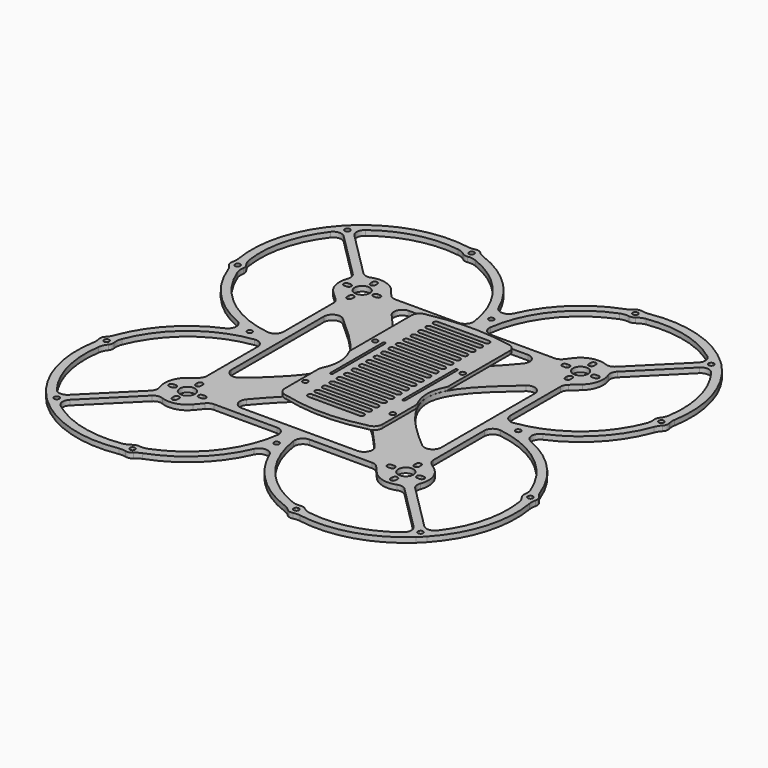
from build123d import *

# Parameters (mm, degrees)
F0_R     = 1.55
F0_R_2   = 4.5
F1_DEPTH = 3
F2_R     = 1.55
F3_DEPTH = 2
F5_DEPTH = 2


# Not quite as in the source:
# - a feature names something its author has since deleted; it is built from what else it names


with BuildPart() as f1:
    # F0 (on Top) → F1 (new body)
    with BuildSketch(Plane.XY):
        with BuildLine():
            ThreePointArc((4.5936412885, 90.9640892891), (1.5876e-06, 87.9385448385), (-4.5936380583, 90.9640893729))
            ThreePointArc((-4.5936380583, 90.9640893729), (-19.7997665524, 112.7493601662), (-42.3857157583, 126.7386155355))
            ThreePointArc((-42.3857157583, 126.7386155355), (-44.282976849, 127.6715883742), (-45.9416856044, 128.9825892242))
            ThreePointArc((-45.9416856044, 128.9825892242), (-47.711537449, 129.9897804476), (-49.7479021723, 129.9951119953))
            ThreePointArc((-49.7479021723, 129.9951119953), (-51.8387697531, 129.6815665856), (-53.9488258268, 129.814612931))
            ThreePointArc((-53.9488258268, 129.814612931), (-83.7536549239, 128.0187505985), (-109.6908840175, 113.2264179235))
            ThreePointArc((-109.6908840175, 113.2264179235), (-111.492270863, 111.492270863), (-113.2264179235, 109.6908840175))
            ThreePointArc((-113.2264179235, 109.6908840175), (-128.0187505985, 83.7536549239), (-129.814612931, 53.9488258268))
            ThreePointArc((-129.814612931, 53.9488258268), (-129.6815665856, 51.8387697531), (-129.9951119953, 49.7479021723))
            ThreePointArc((-129.9951119953, 49.7479021723), (-129.9897804476, 47.711537449), (-128.9825892242, 45.9416856044))
            ThreePointArc((-128.9825892242, 45.9416856044), (-127.6715883742, 44.282976849), (-126.7386155355, 42.3857157583))
            ThreePointArc((-126.7386155355, 42.3857157583), (-112.7493601662, 19.7997665524), (-90.9640893729, 4.5936380583))
            ThreePointArc((-90.9640893729, 4.5936380583), (-87.9385448385, -1.5876e-06), (-90.9640892891, -4.5936412885))
            ThreePointArc((-90.9640892891, -4.5936412885), (-112.7493564136, -19.7997669532), (-126.7386107311, -42.3857113668))
            ThreePointArc((-126.7386107311, -42.3857113668), (-127.6715848934, -44.2829742089), (-128.9825877652, -45.9416841141))
            ThreePointArc((-128.9825877652, -45.9416841141), (-129.9897804476, -47.711537449), (-129.9951114697, -49.7479041907))
            ThreePointArc((-129.9951114697, -49.7479041907), (-129.6815648767, -51.8387737737), (-129.8146109437, -53.9488320249))
            ThreePointArc((-129.8146109437, -53.9488320249), (-128.0187466409, -83.7536577022), (-113.2264144939, -109.6908833036))
            ThreePointArc((-113.2264144939, -109.6908833036), (-111.4922673823, -111.4922701), (-109.6908804846, -113.2264171062))
            ThreePointArc((-109.6908804846, -113.2264171062), (-83.7536558603, -128.018747189), (-53.9488320249, -129.8146109437))
            ThreePointArc((-53.9488320249, -129.8146109437), (-51.8387737737, -129.6815648767), (-49.7479041907, -129.9951114697))
            ThreePointArc((-49.7479041907, -129.9951114697), (-47.711537449, -129.9897804476), (-45.9416841141, -128.9825877652))
            ThreePointArc((-45.9416841141, -128.9825877652), (-44.2829742089, -127.6715848934), (-42.3857113668, -126.7386107311))
            ThreePointArc((-42.3857113668, -126.7386107311), (-19.7997655576, -112.7493550925), (-4.5936397708, -90.9640857581))
            ThreePointArc((-4.5936397708, -90.9640857581), (0, -87.938541039), (4.5936397708, -90.9640857581))
            ThreePointArc((4.5936397708, -90.9640857581), (19.7997655576, -112.7493550925), (42.3857113668, -126.7386107311))
            ThreePointArc((42.3857113668, -126.7386107311), (44.2829742089, -127.6715848934), (45.9416841141, -128.9825877652))
            ThreePointArc((45.9416841141, -128.9825877652), (47.711537449, -129.9897804476), (49.7479041907, -129.9951114697))
            ThreePointArc((49.7479041907, -129.9951114697), (51.8387737737, -129.6815648767), (53.9488320249, -129.8146109437))
            ThreePointArc((53.9488320249, -129.8146109437), (83.7536567813, -128.0187469149), (109.6908818941, -113.2264158001))
            ThreePointArc((109.6908818941, -113.2264158001), (111.4922687411, -111.4922687411), (113.2264158001, -109.6908818941))
            ThreePointArc((113.2264158001, -109.6908818941), (128.0187469149, -83.7536567813), (129.8146109437, -53.9488320249))
            ThreePointArc((129.8146109437, -53.9488320249), (129.6815648767, -51.8387737737), (129.9951114697, -49.7479041907))
            ThreePointArc((129.9951114697, -49.7479041907), (129.9897804476, -47.711537449), (128.9825877652, -45.9416841141))
            ThreePointArc((128.9825877652, -45.9416841141), (127.6715848934, -44.2829742089), (126.7386107311, -42.3857113668))
            ThreePointArc((126.7386107311, -42.3857113668), (112.7493550925, -19.7997655576), (90.9640857581, -4.5936397708))
            ThreePointArc((90.9640857581, -4.5936397708), (87.938541039, 0), (90.9640857581, 4.5936397708))
            ThreePointArc((90.9640857581, 4.5936397708), (112.7493550925, 19.7997655576), (126.7386107311, 42.3857113668))
            ThreePointArc((126.7386107311, 42.3857113668), (127.6715848934, 44.2829742089), (128.9825877652, 45.9416841141))
            ThreePointArc((128.9825877652, 45.9416841141), (129.9897804476, 47.711537449), (129.9951114697, 49.7479041907))
            ThreePointArc((129.9951114697, 49.7479041907), (129.6815648767, 51.8387737737), (129.8146109437, 53.9488320249))
            ThreePointArc((129.8146109437, 53.9488320249), (128.018747189, 83.7536558603), (113.2264171062, 109.6908804846))
            ThreePointArc((113.2264171062, 109.6908804846), (111.4922701, 111.4922673823), (109.6908833036, 113.2264144939))
            ThreePointArc((109.6908833036, 113.2264144939), (83.7536577022, 128.0187466408), (53.9488320249, 129.8146109437))
            ThreePointArc((53.9488320249, 129.8146109437), (51.8387737737, 129.6815648767), (49.7479041907, 129.9951114697))
            ThreePointArc((49.7479041907, 129.9951114697), (47.711537449, 129.9897804476), (45.9416841141, 128.9825877652))
            ThreePointArc((45.9416841141, 128.9825877652), (44.2829742089, 127.6715848934), (42.3857113668, 126.7386107311))
            ThreePointArc((42.3857113668, 126.7386107311), (19.7997669532, 112.7493564136), (4.5936412885, 90.9640892891))
        make_face()
        with Locations((-108.2905437355, -108.153230011)):
            Circle(F0_R, mode=Mode.SUBTRACT)
        with Locations((-48.7398474892, -126.1242172983)):
            Circle(F0_R, mode=Mode.SUBTRACT)
        with BuildLine():
            Line((-66.5, -74.5), (-66.5, -73))
            ThreePointArc((-66.5, -73), (-65, -71.5), (-63.5, -73))
            Line((-63.5, -73), (-63.5, -74.5))
            ThreePointArc((-63.5, -74.5), (-65, -76), (-66.5, -74.5))
        make_face(mode=Mode.SUBTRACT)
        with Locations((-126.1242172983, -48.7398474892)):
            Circle(F0_R, mode=Mode.SUBTRACT)
        with BuildLine():
            Line((-73, -66.5), (-74.5, -66.5))
            ThreePointArc((-74.5, -66.5), (-76, -65), (-74.5, -63.5))
            Line((-74.5, -63.5), (-73, -63.5))
            ThreePointArc((-73, -63.5), (-71.5, -65), (-73, -66.5))
        make_face(mode=Mode.SUBTRACT)
        with Locations((-79.8885448385, 0)):
            Circle(F0_R, mode=Mode.SUBTRACT)
        with Locations((-65, -65)):
            Circle(F0_R_2, mode=Mode.SUBTRACT)
        with BuildLine():
            ThreePointArc((-57, -66.5), (-58.5, -65), (-57, -63.5))
            Line((-57, -63.5), (-55.5, -63.5))
            ThreePointArc((-55.5, -63.5), (-54, -65), (-55.5, -66.5))
            Line((-55.5, -66.5), (-57, -66.5))
        make_face(mode=Mode.SUBTRACT)
        with BuildLine():
            Line((-66.5, -57), (-66.5, -55.5))
            ThreePointArc((-66.5, -55.5), (-65, -54), (-63.5, -55.5))
            Line((-63.5, -55.5), (-63.5, -57))
            ThreePointArc((-63.5, -57), (-65, -58.5), (-66.5, -57))
        make_face(mode=Mode.SUBTRACT)
        with Locations((48.7398474892, -126.1242172983)):
            Circle(F0_R, mode=Mode.SUBTRACT)
        with Locations((0, -79.8885448385)):
            Circle(F0_R, mode=Mode.SUBTRACT)
        with BuildLine():
            ThreePointArc((66.5, -74.5), (65, -76), (63.5, -74.5))
            Line((63.5, -74.5), (63.5, -73))
            ThreePointArc((63.5, -73), (65, -71.5), (66.5, -73))
            Line((66.5, -73), (66.5, -74.5))
        make_face(mode=Mode.SUBTRACT)
        with Locations((108.2784277556, -108.1560280507)):
            Circle(F0_R, mode=Mode.SUBTRACT)
        with BuildLine():
            ThreePointArc((57, -63.5), (58.5, -65), (57, -66.5))
            Line((57, -66.5), (55.5, -66.5))
            ThreePointArc((55.5, -66.5), (54, -65), (55.5, -63.5))
            Line((55.5, -63.5), (57, -63.5))
        make_face(mode=Mode.SUBTRACT)
        with Locations((65, -65)):
            Circle(F0_R_2, mode=Mode.SUBTRACT)
        with BuildLine():
            ThreePointArc((66.5, -57), (65, -58.5), (63.5, -57))
            Line((63.5, -57), (63.5, -55.5))
            ThreePointArc((63.5, -55.5), (65, -54), (66.5, -55.5))
            Line((66.5, -55.5), (66.5, -57))
        make_face(mode=Mode.SUBTRACT)
        with BuildLine():
            ThreePointArc((-78.7260276961, 75.1904937901), (-77.3700677078, 72.6909557736), (-77.5962746825, 69.8563220777))
            ThreePointArc((-77.5962746825, 69.8563220777), (-78.1774623607, 62.066659629), (-74.3468847944, 55.2590685948))
            ThreePointArc((-74.3468847944, 55.2590685948), (-55.8574100489, 55.0670724866), (-54.5192604238, 73.5090597562))
            ThreePointArc((-54.5192604238, 73.5090597562), (-61.5236729853, 78.0447365051), (-69.8563220777, 77.5962746825))
            ThreePointArc((-69.8563220777, 77.5962746825), (-72.6909557736, 77.3700677078), (-75.1904937901, 78.7260276961))
            Line((-75.1904937901, 78.7260276961), (-102.2950830455, 105.8306169514))
            ThreePointArc((-102.2950830455, 105.8306169514), (-103.7481732445, 109.7032406669), (-101.7873113942, 113.3451778401))
            ThreePointArc((-101.7873113942, 113.3451778401), (-80.0827992563, 123.8478688365), (-56.0022199647, 125.0799671641))
            ThreePointArc((-56.0022199647, 125.0799671641), (-53.4825995412, 124.3550905641), (-51.2379870694, 123.0002296802))
            ThreePointArc((-51.2379870694, 123.0002296802), (-49.7681575294, 122.258654149), (-48.1241365653, 122.1718888632))
            ThreePointArc((-48.1241365653, 122.1718888632), (-45.5030157293, 122.2323762703), (-42.9562600942, 121.6095047758))
            ThreePointArc((-42.9562600942, 121.6095047758), (-17.2773803845, 102.5914096175), (-4.8022395632, 73.1726457399))
            ThreePointArc((-4.8022395632, 73.1726457399), (-5.9909393236, 69.2108685569), (-9.7567877473, 67.5))
            Line((-9.7567877473, 67.5), (-47.2749619701, 67.5))
            ThreePointArc((-47.2749619701, 67.5), (-49.4332948043, 67.989833775), (-51.1687379105, 69.3633602493))
            add(Edge.make_bspline(
                [(-51.1687379105, 69.3633602493), (-47.007111135, 64.1971813129), (-42.9204896878, 59.0857782526), (-38.8861434054, 54.2837422746)],
                knots=[0.0293673697, 0.0293673697, 0.0293673697, 0.0293673697, 0.1393383892, 0.1393383892, 0.1393383892, 0.1393383892], degree=3))
            ThreePointArc((-38.8861434054, 54.2837422746), (-39.5900475875, 59.6117186571), (-35.0578688274, 62.5))
            Line((-35.0578688274, 62.5), (35.6142056633, 62.5))
            ThreePointArc((35.6142056633, 62.5), (40.1396288907, 59.6261572409), (39.4629102085, 54.3082178452))
            add(Edge.make_bspline(
                [(39.4629102085, 54.3082178452), (43.4572386204, 59.1246461501), (47.4477718972, 64.2594353508), (51.4265936274, 69.4628891406)],
                knots=[0.8640600007, 0.8640600007, 0.8640600007, 0.8640600007, 0.9739367654, 0.9739367654, 0.9739367654, 0.9739367654], degree=3))
            ThreePointArc((51.4265936274, 69.4628891406), (49.6699228907, 68.0175032461), (47.4546976535, 67.5))
            Line((47.4546976535, 67.5), (9.7567877473, 67.5))
            ThreePointArc((9.7567877473, 67.5), (5.9909393236, 69.2108685569), (4.8022395632, 73.1726457399))
            ThreePointArc((4.8022395632, 73.1726457399), (17.2773803845, 102.5914096175), (42.9562600942, 121.6095047758))
            ThreePointArc((42.9562600942, 121.6095047758), (45.5030157293, 122.2323762703), (48.1241365653, 122.1718888632))
            ThreePointArc((48.1241365653, 122.1718888632), (49.7681575294, 122.258654149), (51.2379870694, 123.0002296802))
            ThreePointArc((51.2379870694, 123.0002296802), (53.4825995412, 124.3550905641), (56.0022199647, 125.0799671641))
            ThreePointArc((56.0022199647, 125.0799671641), (80.0828001163, 123.8478686161), (101.7873128072, 113.3451767649))
            ThreePointArc((101.7873128072, 113.3451767649), (103.748174551, 109.7032395344), (102.2950842388, 105.8306158614))
            Line((102.2950842388, 105.8306158614), (75.1904941913, 78.7260273982))
            ThreePointArc((75.1904941913, 78.7260273982), (72.6909561352, 77.370067483), (69.8563224458, 77.5962745406))
            ThreePointArc((69.8563224458, 77.5962745406), (61.3181994895, 77.9882387182), (54.2558912586, 73.1739909073))
            ThreePointArc((54.2558912586, 73.1739909073), (55.8750675797, 55.0508488641), (74.0703287451, 55.0010432317))
            ThreePointArc((74.0703287451, 55.0010432317), (78.1350771686, 61.8823489971), (77.5962748245, 69.8563217095))
            ThreePointArc((77.5962748245, 69.8563217095), (77.3700679326, 72.6909554121), (78.7260279939, 75.190493389))
            Line((78.7260279939, 75.190493389), (105.8306180414, 102.2950818521))
            ThreePointArc((105.8306180414, 102.2950818521), (109.7032417994, 103.7481719379), (113.3451789152, 101.7873099812))
            ThreePointArc((113.3451789152, 101.7873099812), (123.8478690569, 80.0827983963), (125.0799671641, 56.0022199647))
            ThreePointArc((125.0799671641, 56.0022199647), (124.3550905641, 53.4825995412), (123.0002296802, 51.2379870694))
            ThreePointArc((123.0002296802, 51.2379870694), (122.258654149, 49.7681575294), (122.1718888632, 48.1241365653))
            ThreePointArc((122.1718888632, 48.1241365653), (122.2323762703, 45.5030157293), (121.6095047758, 42.9562600942))
            ThreePointArc((121.6095047758, 42.9562600942), (102.5914096175, 17.2773803845), (73.1726457399, 4.8022395632))
            ThreePointArc((73.1726457399, 4.8022395632), (69.2108685569, 5.9909393236), (67.5, 9.7567877473))
            Line((67.5, 9.7567877473), (67.5, 46.9024650002))
            ThreePointArc((67.5, 46.9024650002), (67.9450696625, 48.9646506418), (69.2010438482, 50.6597097764))
            add(Edge.make_bspline(
                [(69.2010438482, 50.6597097764), (64.0951140729, 46.1765740091), (59.0182901872, 41.9052788751), (54.2353248312, 37.7820833857)],
                knots=[0.0348728398, 0.0348728398, 0.0348728398, 0.0348728398, 0.1445829675, 0.1445829675, 0.1445829675, 0.1445829675], degree=3))
            ThreePointArc((54.2353248312, 37.7820833857), (59.5828615119, 38.5405267444), (62.5, 33.9950138006))
            Line((62.5, 33.9950138006), (62.5, -35.5495988309))
            ThreePointArc((62.5, -35.5495988309), (59.6206264771, -40.0776164264), (54.2988226622, -39.3904924316))
            add(Edge.make_bspline(
                [(54.2988226622, -39.3904924316), (59.1121784473, -43.4021644694), (64.2467475497, -47.4153572737), (69.4560669959, -51.4128712838)],
                knots=[0.8650150287, 0.8650150287, 0.8650150287, 0.8650150287, 0.9740421792, 0.9740421792, 0.9740421792, 0.9740421792], degree=3))
            ThreePointArc((69.4560669959, -51.4128712838), (68.0156012097, -49.6575734697), (67.5, -47.4462011605))
            Line((67.5, -47.4462011605), (67.5, -9.7567877473))
            ThreePointArc((67.5, -9.7567877473), (69.2108685569, -5.9909393236), (73.1726457399, -4.8022395632))
            ThreePointArc((73.1726457399, -4.8022395632), (102.5914096175, -17.2773803845), (121.6095047758, -42.9562600942))
            ThreePointArc((121.6095047758, -42.9562600942), (122.2323762703, -45.5030157293), (122.1718888632, -48.1241365653))
            ThreePointArc((122.1718888632, -48.1241365653), (122.258654149, -49.7681575294), (123.0002296802, -51.2379870694))
            ThreePointArc((123.0002296802, -51.2379870694), (124.3550905641, -53.4825995412), (125.0799671641, -56.0022199647))
            ThreePointArc((125.0799671641, -56.0022199647), (123.8478688365, -80.0827992563), (113.3451778401, -101.7873113942))
            ThreePointArc((113.3451778401, -101.7873113942), (109.7032406669, -103.7481732445), (105.8306169514, -102.2950830455))
            Line((105.8306169514, -102.2950830455), (78.7260276961, -75.1904937901))
            ThreePointArc((78.7260276961, -75.1904937901), (77.3700677078, -72.6909557736), (77.5962746825, -69.8563220777))
            ThreePointArc((77.5962746825, -69.8563220777), (77.9903375994, -61.3256117442), (73.1862480092, -54.2652273647))
            ThreePointArc((73.1862480092, -54.2652273647), (55.0961710642, -55.8258966427), (54.9219208197, -73.9823337745))
            ThreePointArc((54.9219208197, -73.9823337745), (61.8248103944, -78.1212869403), (69.8563220777, -77.5962746825))
            ThreePointArc((69.8563220777, -77.5962746825), (72.6909557736, -77.3700677078), (75.1904937901, -78.7260276961))
            Line((75.1904937901, -78.7260276961), (102.2950830455, -105.8306169514))
            ThreePointArc((102.2950830455, -105.8306169514), (103.7481732445, -109.7032406669), (101.7873113942, -113.3451778401))
            ThreePointArc((101.7873113942, -113.3451778401), (80.0827992563, -123.8478688365), (56.0022199647, -125.0799671641))
            ThreePointArc((56.0022199647, -125.0799671641), (53.4825995412, -124.3550905641), (51.2379870694, -123.0002296802))
            ThreePointArc((51.2379870694, -123.0002296802), (49.7681575294, -122.258654149), (48.1241365653, -122.1718888632))
            ThreePointArc((48.1241365653, -122.1718888632), (45.5030157293, -122.2323762703), (42.9562600942, -121.6095047758))
            ThreePointArc((42.9562600942, -121.6095047758), (17.2773803845, -102.5914096175), (4.8022395632, -73.1726457399))
            ThreePointArc((4.8022395632, -73.1726457399), (5.9909393236, -69.2108685569), (9.7567877473, -67.5))
            Line((9.7567877473, -67.5), (46.9610754937, -67.5))
            ThreePointArc((46.9610754937, -67.5), (49.0351777215, -67.9504835478), (50.7355403773, -69.2207600206))
            add(Edge.make_bspline(
                [(50.7355403773, -69.2207600206), (46.2776004608, -64.0895900624), (42.0082462932, -59.0081310929), (37.8793761718, -54.2306155101)],
                knots=[0.0336445481, 0.0336445481, 0.0336445481, 0.0336445481, 0.1425668185, 0.1425668185, 0.1425668185, 0.1425668185], degree=3))
            ThreePointArc((37.8793761718, -54.2306155101), (38.6431792121, -59.5800333592), (34.0963714061, -62.5))
            Line((34.0963714061, -62.5), (-34.6716965747, -62.5))
            ThreePointArc((-34.6716965747, -62.5), (-39.2116462302, -59.594959934), (-38.4761016269, -54.25554285))
            add(Edge.make_bspline(
                [(-38.4761016269, -54.25554285), (-42.5524815665, -59.0354489236), (-46.7247402937, -64.1334390375), (-51.0163929038, -69.3081210856)],
                knots=[0.86152407, 0.86152407, 0.86152407, 0.86152407, 0.9696650908, 0.9696650908, 0.9696650908, 0.9696650908], degree=3))
            ThreePointArc((-51.0163929038, -69.3081210856), (-49.2938689584, -67.974550046), (-47.1677686047, -67.5))
            Line((-47.1677686047, -67.5), (-9.7567877474, -67.5))
            ThreePointArc((-9.7567877474, -67.5), (-5.9909393237, -69.2108685569), (-4.8022395633, -73.1726457399))
            ThreePointArc((-4.8022395633, -73.1726457399), (-17.2773803846, -102.5914096175), (-42.9562600944, -121.6095047758))
            ThreePointArc((-42.9562600944, -121.6095047758), (-45.5030157294, -122.2323762703), (-48.1241365654, -122.1718888632))
            ThreePointArc((-48.1241365654, -122.1718888632), (-49.7681575294, -122.258654149), (-51.2379870693, -123.0002296802))
            ThreePointArc((-51.2379870693, -123.0002296802), (-53.4825995411, -124.355090564), (-56.0022199645, -125.079967164))
            ThreePointArc((-56.0022199645, -125.079967164), (-80.0827983962, -123.8478690568), (-101.7873099811, -113.3451789152))
            ThreePointArc((-101.7873099811, -113.3451789152), (-103.7481719378, -109.7032417994), (-102.295081852, -105.8306180414))
            Line((-102.295081852, -105.8306180414), (-75.190493389, -78.7260279939))
            ThreePointArc((-75.190493389, -78.7260279939), (-72.6909554121, -77.3700679326), (-69.8563217095, -77.5962748245))
            ThreePointArc((-69.8563217095, -77.5962748245), (-61.6280970797, -78.0721180647), (-54.6566830252, -73.6755860873))
            ThreePointArc((-54.6566830252, -73.6755860873), (-55.3115936341, -55.5986818962), (-73.3606290294, -54.4004772639))
            ThreePointArc((-73.3606290294, -54.4004772639), (-78.019936228, -61.431910789), (-77.5962745406, -69.8563224458))
            ThreePointArc((-77.5962745406, -69.8563224458), (-77.370067483, -72.6909561352), (-78.7260273982, -75.1904941913))
            Line((-78.7260273982, -75.1904941913), (-105.8306158613, -102.2950842388))
            ThreePointArc((-105.8306158613, -102.2950842388), (-109.7032395344, -103.7481745509), (-113.3451767648, -101.7873128071))
            ThreePointArc((-113.3451767648, -101.7873128071), (-123.847868616, -80.0828001162), (-125.079967164, -56.0022199645))
            ThreePointArc((-125.079967164, -56.0022199645), (-124.355090564, -53.4825995411), (-123.0002296802, -51.2379870693))
            ThreePointArc((-123.0002296802, -51.2379870693), (-122.258654149, -49.7681575294), (-122.1718888632, -48.1241365654))
            ThreePointArc((-122.1718888632, -48.1241365654), (-122.2323762703, -45.5030157294), (-121.6095047758, -42.9562600944))
            ThreePointArc((-121.6095047758, -42.9562600944), (-102.5915462524, -17.277488013), (-73.1729904451, -4.8022863626))
            ThreePointArc((-73.1729904451, -4.8022863626), (-69.2111956733, -5.9909728541), (-67.5003163344, -9.7568306947))
            Line((-67.5003163344, -9.7568306947), (-67.5003163328, -47.353236691))
            ThreePointArc((-67.5003163328, -47.353236691), (-68.0006204029, -49.5333138774), (-69.4014109482, -51.2771104681))
            add(Edge.make_bspline(
                [(-54.2790618736, -39.0485616103), (-59.0828616964, -43.094423634), (-64.2057413604, -47.1737958924), (-69.4014109482, -51.2771104681)],
                knots=[0.8641405018, 0.8641405018, 0.8641405018, 0.8641405018, 0.9725362801, 0.9725362801, 0.9725362801, 0.9725362801], degree=3))
            ThreePointArc((-54.2790618736, -39.0485616103), (-59.6089463445, -39.7576935316), (-62.5, -35.2242240748))
            Line((-62.5, -35.2242240748), (-62.5, 33.4095018987))
            ThreePointArc((-62.5, 33.4095018987), (-59.5674116994, 37.9620625919), (-54.209676454, 37.1743087945))
            add(Edge.make_bspline(
                [(-69.1233391423, 50.3680202269), (-64.0476785875, 45.7195000527), (-58.9859996351, 41.3486659558), (-54.209676454, 37.1743087945)],
                knots=[0.0376140132, 0.0376140132, 0.0376140132, 0.0376140132, 0.147134592, 0.147134592, 0.147134592, 0.147134592], degree=3))
            ThreePointArc((-69.1233391423, 50.3680202269), (-67.9240249358, 48.6950792761), (-67.5003163367, 46.6807414163))
            Line((-67.5003163367, 46.6807414163), (-67.5003163352, 9.7568306951))
            ThreePointArc((-67.5003163352, 9.7568306951), (-69.211195674, 5.9909728542), (-73.1729904459, 4.8022863626))
            ThreePointArc((-73.1729904459, 4.8022863626), (-102.5915462527, 17.2774880132), (-121.6095047758, 42.9562600942))
            ThreePointArc((-121.6095047758, 42.9562600942), (-122.2323762703, 45.5030157293), (-122.1718888632, 48.1241365653))
            ThreePointArc((-122.1718888632, 48.1241365653), (-122.258654149, 49.7681575294), (-123.0002296802, 51.2379870694))
            ThreePointArc((-123.0002296802, 51.2379870694), (-124.3550905641, 53.4825995412), (-125.0799671641, 56.0022199647))
            ThreePointArc((-125.0799671641, 56.0022199647), (-123.8478688365, 80.0827992563), (-113.3451778401, 101.7873113942))
            ThreePointArc((-113.3451778401, 101.7873113942), (-109.7032406669, 103.7481732445), (-105.8306169514, 102.2950830455))
            Line((-105.8306169514, 102.2950830455), (-78.7260276961, 75.1904937901))
        make_face(mode=Mode.SUBTRACT)
        with BuildLine():
            ThreePointArc((74.5, -63.5), (76, -65), (74.5, -66.5))
            Line((74.5, -66.5), (73, -66.5))
            ThreePointArc((73, -66.5), (71.5, -65), (73, -63.5))
            Line((73, -63.5), (74.5, -63.5))
        make_face(mode=Mode.SUBTRACT)
        with Locations((126.1242172983, -48.7398474892)):
            Circle(F0_R, mode=Mode.SUBTRACT)
        with Locations((79.8885448385, 0)):
            Circle(F0_R, mode=Mode.SUBTRACT)
        with Locations((-126.1242172983, 48.7398474892)):
            Circle(F0_R, mode=Mode.SUBTRACT)
        with BuildLine():
            ThreePointArc((-73, 66.5), (-71.5, 65), (-73, 63.5))
            Line((-73, 63.5), (-74.5, 63.5))
            ThreePointArc((-74.5, 63.5), (-76, 65), (-74.5, 66.5))
            Line((-74.5, 66.5), (-73, 66.5))
        make_face(mode=Mode.SUBTRACT)
        with BuildLine():
            ThreePointArc((-63.5, 55.5), (-65, 54), (-66.5, 55.5))
            Line((-66.5, 55.5), (-66.5, 57))
            ThreePointArc((-66.5, 57), (-65, 58.5), (-63.5, 57))
            Line((-63.5, 57), (-63.5, 55.5))
        make_face(mode=Mode.SUBTRACT)
        with Locations((-65, 65)):
            Circle(F0_R_2, mode=Mode.SUBTRACT)
        with BuildLine():
            Line((-55.5, 63.5), (-57, 63.5))
            ThreePointArc((-57, 63.5), (-58.5, 65), (-57, 66.5))
            Line((-57, 66.5), (-55.5, 66.5))
            ThreePointArc((-55.5, 66.5), (-54, 65), (-55.5, 63.5))
        make_face(mode=Mode.SUBTRACT)
        with Locations((-108.3014905595, 108.1507019099)):
            Circle(F0_R, mode=Mode.SUBTRACT)
        with BuildLine():
            ThreePointArc((-63.5, 73), (-65, 71.5), (-66.5, 73))
            Line((-66.5, 73), (-66.5, 74.5))
            ThreePointArc((-66.5, 74.5), (-65, 76), (-63.5, 74.5))
            Line((-63.5, 74.5), (-63.5, 73))
        make_face(mode=Mode.SUBTRACT)
        with Locations((-48.7398474892, 126.1242172983)):
            Circle(F0_R, mode=Mode.SUBTRACT)
        with BuildLine():
            Line((63.5, 55.5), (63.5, 57))
            ThreePointArc((63.5, 57), (65, 58.5), (66.5, 57))
            Line((66.5, 57), (66.5, 55.5))
            ThreePointArc((66.5, 55.5), (65, 54), (63.5, 55.5))
        make_face(mode=Mode.SUBTRACT)
        with BuildLine():
            Line((55.5, 66.5), (57, 66.5))
            ThreePointArc((57, 66.5), (58.5, 65), (57, 63.5))
            Line((57, 63.5), (55.5, 63.5))
            ThreePointArc((55.5, 63.5), (54, 65), (55.5, 66.5))
        make_face(mode=Mode.SUBTRACT)
        with Locations((65, 65)):
            Circle(F0_R_2, mode=Mode.SUBTRACT)
        with BuildLine():
            Line((74.5, 63.5), (73, 63.5))
            ThreePointArc((73, 63.5), (71.5, 65), (73, 66.5))
            Line((73, 66.5), (74.5, 66.5))
            ThreePointArc((74.5, 66.5), (76, 65), (74.5, 63.5))
        make_face(mode=Mode.SUBTRACT)
        with Locations((126.1242172983, 48.7398474892)):
            Circle(F0_R, mode=Mode.SUBTRACT)
        with Locations((0, 79.8885448385)):
            Circle(F0_R, mode=Mode.SUBTRACT)
        with BuildLine():
            Line((66.5, 74.5), (66.5, 73))
            ThreePointArc((66.5, 73), (65, 71.5), (63.5, 73))
            Line((63.5, 73), (63.5, 74.5))
            ThreePointArc((63.5, 74.5), (65, 76), (66.5, 74.5))
        make_face(mode=Mode.SUBTRACT)
        with Locations((48.7398474892, 126.1242172983)):
            Circle(F0_R, mode=Mode.SUBTRACT)
        with Locations((108.153230011, 108.2905437356)):
            Circle(F0_R, mode=Mode.SUBTRACT)
        with BuildLine():
            ThreePointArc((-54.5192604238, 73.5090597562), (-55.8574100489, 55.0670724866), (-74.3468847944, 55.2590685948))
            add(Edge.make_bspline(
                [(-74.3468847944, 55.2590685948), (-72.6113826473, 53.5937721304), (-70.8665363109, 51.9645192675), (-69.1233391423, 50.3680202269)],
                knots=[0, 0, 0, 0, 0.0376140132, 0.0376140132, 0.0376140132, 0.0376140132], degree=3))
            add(Edge.make_bspline(
                [(-69.1233391423, 50.3680202269), (-64.0476785875, 45.7195000527), (-58.9859996351, 41.3486659558), (-54.209676454, 37.1743087945)],
                knots=[0.0376140132, 0.0376140132, 0.0376140132, 0.0376140132, 0.147134592, 0.147134592, 0.147134592, 0.147134592], degree=3))
            add(Edge.make_bspline(
                [(-54.209676454, 37.1743087945), (-38.7237596273, 23.6401015491), (-13.5112663594, 0.4819895204), (-38.2399723309, -25.540100461), (-54.2790618736, -39.0485616103)],
                knots=[0.147134592, 0.147134592, 0.147134592, 0.147134592, 0.5022250058, 0.8641405018, 0.8641405018, 0.8641405018, 0.8641405018], degree=3))
            add(Edge.make_bspline(
                [(-54.2790618736, -39.0485616103), (-59.0828616964, -43.094423634), (-64.2057413604, -47.1737958924), (-69.4014109482, -51.2771104681)],
                knots=[0.8641405018, 0.8641405018, 0.8641405018, 0.8641405018, 0.9725362801, 0.9725362801, 0.9725362801, 0.9725362801], degree=3))
            add(Edge.make_bspline(
                [(-69.4014109482, -51.2771104681), (-70.7178128987, -52.3167476543), (-72.0388875207, -53.3579217921), (-73.3606290294, -54.4004772639)],
                knots=[0.9725362801, 0.9725362801, 0.9725362801, 0.9725362801, 1, 1, 1, 1], degree=3))
            ThreePointArc((-73.3606290294, -54.4004772639), (-55.3115936341, -55.5986818962), (-54.6566830252, -73.6755860873))
            add(Edge.make_bspline(
                [(-51.0163929038, -69.3081210856), (-52.2202551514, -70.7596841376), (-53.4335121775, -72.2172818685), (-54.6566830252, -73.6755860873)],
                knots=[0.9696650908, 0.9696650908, 0.9696650908, 0.9696650908, 1, 1, 1, 1], degree=3))
            add(Edge.make_bspline(
                [(-38.4761016269, -54.25554285), (-42.5524815665, -59.0354489236), (-46.7247402937, -64.1334390375), (-51.0163929038, -69.3081210856)],
                knots=[0.86152407, 0.86152407, 0.86152407, 0.86152407, 0.9696650908, 0.9696650908, 0.9696650908, 0.9696650908], degree=3))
            add(Edge.make_bspline(
                [(37.8793761718, -54.2306155101), (24.3041480834, -38.5227192032), (0.0997442999, -13.5842522629), (-24.8744525972, -38.3064395346), (-38.4761016269, -54.25554285)],
                knots=[0.1425668185, 0.1425668185, 0.1425668185, 0.1425668185, 0.500690136, 0.86152407, 0.86152407, 0.86152407, 0.86152407], degree=3))
            add(Edge.make_bspline(
                [(50.7355403773, -69.2207600206), (46.2776004608, -64.0895900624), (42.0082462932, -59.0081310929), (37.8793761718, -54.2306155101)],
                knots=[0.0336445481, 0.0336445481, 0.0336445481, 0.0336445481, 0.1425668185, 0.1425668185, 0.1425668185, 0.1425668185], degree=3))
            add(Edge.make_bspline(
                [(54.9219208197, -73.9823337745), (53.5075225493, -72.3953945536), (52.112534936, -70.8057058127), (50.7355403773, -69.2207600206)],
                knots=[0, 0, 0, 0, 0.0336445481, 0.0336445481, 0.0336445481, 0.0336445481], degree=3))
            ThreePointArc((54.9219208197, -73.9823337745), (55.0961710642, -55.8258966427), (73.1862480092, -54.2652273647))
            add(Edge.make_bspline(
                [(69.4560669959, -51.4128712838), (70.6963321973, -52.3646227688), (71.940834612, -53.3154855034), (73.1862480092, -54.2652273647)],
                knots=[0.9740421792, 0.9740421792, 0.9740421792, 0.9740421792, 1, 1, 1, 1], degree=3))
            add(Edge.make_bspline(
                [(54.2988226622, -39.3904924316), (59.1121784473, -43.4021644694), (64.2467475497, -47.4153572737), (69.4560669959, -51.4128712838)],
                knots=[0.8650150287, 0.8650150287, 0.8650150287, 0.8650150287, 0.9740421792, 0.9740421792, 0.9740421792, 0.9740421792], degree=3))
            add(Edge.make_bspline(
                [(54.2353248312, 37.7820833857), (38.6550415809, 24.3509692464), (13.5326368893, 0.4431862355), (38.2705199865, -26.0317679723), (54.2988226622, -39.3904924316)],
                knots=[0.1445829675, 0.1445829675, 0.1445829675, 0.1445829675, 0.5019585155, 0.8650150287, 0.8650150287, 0.8650150287, 0.8650150287], degree=3))
            add(Edge.make_bspline(
                [(69.2010438482, 50.6597097764), (64.0951140729, 46.1765740091), (59.0182901872, 41.9052788751), (54.2353248312, 37.7820833857)],
                knots=[0.0348728398, 0.0348728398, 0.0348728398, 0.0348728398, 0.1445829675, 0.1445829675, 0.1445829675, 0.1445829675], degree=3))
            add(Edge.make_bspline(
                [(74.0703287451, 55.0010432317), (72.4499615375, 53.5311635631), (70.8240323045, 52.0847347804), (69.2010438482, 50.6597097764)],
                knots=[0, 0, 0, 0, 0.0348728398, 0.0348728398, 0.0348728398, 0.0348728398], degree=3))
            ThreePointArc((74.0703287451, 55.0010432317), (55.8750675797, 55.0508488641), (54.2558912586, 73.1739909073))
            add(Edge.make_bspline(
                [(51.4265936274, 69.4628891406), (52.3703870168, 70.6971704484), (53.3135214459, 71.9353152278), (54.2558912586, 73.1739909073)],
                knots=[0.9739367654, 0.9739367654, 0.9739367654, 0.9739367654, 1, 1, 1, 1], degree=3))
            add(Edge.make_bspline(
                [(39.4629102085, 54.3082178452), (43.4572386204, 59.1246461501), (47.4477718972, 64.2594353508), (51.4265936274, 69.4628891406)],
                knots=[0.8640600007, 0.8640600007, 0.8640600007, 0.8640600007, 0.9739367654, 0.9739367654, 0.9739367654, 0.9739367654], degree=3))
            add(Edge.make_bspline(
                [(-38.8861434054, 54.2837422746), (-25.628452755, 38.5032655801), (-0.1737443139, 13.5570975552), (26.2546916853, 38.3815260478), (39.4629102085, 54.3082178452)],
                knots=[0.1393383892, 0.1393383892, 0.1393383892, 0.1393383892, 0.5007257504, 0.8640600007, 0.8640600007, 0.8640600007, 0.8640600007], degree=3))
            add(Edge.make_bspline(
                [(-51.1687379105, 69.3633602493), (-47.007111135, 64.1971813129), (-42.9204896878, 59.0857782526), (-38.8861434054, 54.2837422746)],
                knots=[0.0293673697, 0.0293673697, 0.0293673697, 0.0293673697, 0.1393383892, 0.1393383892, 0.1393383892, 0.1393383892], degree=3))
            add(Edge.make_bspline(
                [(-54.5192604238, 73.5090597562), (-53.3967820872, 72.126485951), (-52.2800855412, 70.7429699621), (-51.1687379105, 69.3633602493)],
                knots=[0, 0, 0, 0, 0.0293673697, 0.0293673697, 0.0293673697, 0.0293673697], degree=3))
        make_face()
        with Locations((-26, -26)):
            Circle(F0_R, mode=Mode.SUBTRACT)
        with Locations((-15.25, -15.25)):
            Circle(F0_R, mode=Mode.SUBTRACT)
        with Locations((26, -26)):
            Circle(F0_R, mode=Mode.SUBTRACT)
        with Locations((15.25, -15.25)):
            Circle(F0_R, mode=Mode.SUBTRACT)
        with Locations((-15.25, 15.25)):
            Circle(F0_R, mode=Mode.SUBTRACT)
        with Locations((-26, 26)):
            Circle(F0_R, mode=Mode.SUBTRACT)
        with Locations((15.25, 15.25)):
            Circle(F0_R, mode=Mode.SUBTRACT)
        with Locations((26, 26)):
            Circle(F0_R, mode=Mode.SUBTRACT)
    extrude(amount=F1_DEPTH)


with BuildPart() as f3:
    # F2 (on face) → F3 (new body)
    with BuildSketch(Plane.XY.offset(3)):
        with BuildLine():
            ThreePointArc((24, -42.5), (27.5355339059, -41.0355339059), (29, -37.5))
            Line((29, -37.5), (29, -12.875568205))
            ThreePointArc((29, -12.875568205), (28.8569327081, -11.6880478183), (28.4359181325, -10.568485562))
            ThreePointArc((28.4359181325, -10.568485562), (25.9619697959, -0.4500903501), (28.4359181325, 9.6683048618))
            ThreePointArc((28.4359181325, 9.6683048618), (28.8569327081, 10.7878671182), (29, 11.9753875048))
            Line((29, 11.9753875048), (29, 56.9753875048))
            ThreePointArc((29, 56.9753875048), (27.5355339059, 60.5109214108), (24, 61.9753875048))
            ThreePointArc((24, 61.9753875048), (-0.0190194291, 64.2433746937), (-24, 61.6033688072))
            ThreePointArc((-24, 61.6033688072), (-27.5355339059, 60.1389027131), (-29, 56.6033688072))
            Line((-29, 56.6033688072), (-29, 11.6033688072))
            ThreePointArc((-29, 11.6033688072), (-28.864053581, 10.4453607066), (-28.4636068956, 9.3503234278))
            ThreePointArc((-28.4636068956, 9.3503234278), (-26.111095842, -0.531075337), (-28.4636068956, -10.4124741017))
            ThreePointArc((-28.4636068956, -10.4124741017), (-28.864053581, -11.5075113805), (-29, -12.6655194811))
            Line((-29, -12.6655194811), (-29, -37.5))
            ThreePointArc((-29, -37.5), (-27.5355339059, -41.0355339059), (-24, -42.5))
            ThreePointArc((-24, -42.5), (0, -45.548100799), (24, -42.5))
        make_face()
        with Locations((-26, -26)):
            Circle(F2_R, mode=Mode.SUBTRACT)
        with Locations((26, -26)):
            Circle(F2_R, mode=Mode.SUBTRACT)
        with Locations((-26, 26)):
            Circle(F2_R, mode=Mode.SUBTRACT)
        with Locations((26, 26)):
            Circle(F2_R, mode=Mode.SUBTRACT)
    extrude(amount=F3_DEPTH)

    # F4 (on face) → F5 (cut, through all)
    with BuildSketch(Plane.XY.offset(5)):
        with BuildLine():
            ThreePointArc((-15.293141827, 37.25), (-16.793141827, 35.75), (-15.293141827, 34.25))
            Line((-15.293141827, 34.25), (15.288121067, 34.25))
            ThreePointArc((15.288121067, 34.25), (16.788121067, 35.75), (15.288121067, 37.25))
            Line((15.288121067, 37.25), (-15.293141827, 37.25))
        make_face()
        with BuildLine():
            ThreePointArc((-15.293141827, 31.75), (-16.793141827, 30.25), (-15.293141827, 28.75))
            Line((-15.293141827, 28.75), (15.288121067, 28.75))
            ThreePointArc((15.288121067, 28.75), (16.788121067, 30.25), (15.288121067, 31.75))
            Line((15.288121067, 31.75), (-15.293141827, 31.75))
        make_face()
        with BuildLine():
            ThreePointArc((-15.293141827, 26.25), (-16.793141827, 24.75), (-15.293141827, 23.25))
            Line((-15.293141827, 23.25), (15.288121067, 23.25))
            ThreePointArc((15.288121067, 23.25), (16.788121067, 24.75), (15.288121067, 26.25))
            Line((15.288121067, 26.25), (-15.293141827, 26.25))
        make_face()
        with BuildLine():
            ThreePointArc((-15.293141827, 20.75), (-16.793141827, 19.25), (-15.293141827, 17.75))
            Line((-15.293141827, 17.75), (15.288121067, 17.75))
            ThreePointArc((15.288121067, 17.75), (16.788121067, 19.25), (15.288121067, 20.75))
            Line((15.288121067, 20.75), (-15.293141827, 20.75))
        make_face()
        with BuildLine():
            ThreePointArc((-15.293141827, 15.25), (-16.793141827, 13.75), (-15.293141827, 12.25))
            Line((-15.293141827, 12.25), (15.288121067, 12.25))
            ThreePointArc((15.288121067, 12.25), (16.788121067, 13.75), (15.288121067, 15.25))
            Line((15.288121067, 15.25), (-15.293141827, 15.25))
        make_face()
        with BuildLine():
            ThreePointArc((-15.293141827, 9.75), (-16.793141827, 8.25), (-15.293141827, 6.75))
            Line((-15.293141827, 6.75), (15.288121067, 6.75))
            ThreePointArc((15.288121067, 6.75), (16.788121067, 8.25), (15.288121067, 9.75))
            Line((15.288121067, 9.75), (-15.293141827, 9.75))
        make_face()
        with BuildLine():
            ThreePointArc((-15.293141827, 4.25), (-16.793141827, 2.75), (-15.293141827, 1.25))
            Line((-15.293141827, 1.25), (15.288121067, 1.25))
            ThreePointArc((15.288121067, 1.25), (16.788121067, 2.75), (15.288121067, 4.25))
            Line((15.288121067, 4.25), (-15.293141827, 4.25))
        make_face()
        with BuildLine():
            ThreePointArc((-15.293141827, -1.25), (-16.793141827, -2.75), (-15.293141827, -4.25))
            Line((-15.293141827, -4.25), (15.288121067, -4.25))
            ThreePointArc((15.288121067, -4.25), (16.788121067, -2.75), (15.288121067, -1.25))
            Line((15.288121067, -1.25), (-15.293141827, -1.25))
        make_face()
        with BuildLine():
            ThreePointArc((-15.293141827, -6.75), (-16.793141827, -8.25), (-15.293141827, -9.75))
            Line((-15.293141827, -9.75), (15.288121067, -9.75))
            ThreePointArc((15.288121067, -9.75), (16.788121067, -8.25), (15.288121067, -6.75))
            Line((15.288121067, -6.75), (-15.293141827, -6.75))
        make_face()
        with BuildLine():
            ThreePointArc((-15.293141827, -12.25), (-16.793141827, -13.75), (-15.293141827, -15.25))
            Line((-15.293141827, -15.25), (15.288121067, -15.25))
            ThreePointArc((15.288121067, -15.25), (16.788121067, -13.75), (15.288121067, -12.25))
            Line((15.288121067, -12.25), (-15.293141827, -12.25))
        make_face()
        with BuildLine():
            ThreePointArc((-15.293141827, -17.75), (-16.793141827, -19.25), (-15.293141827, -20.75))
            Line((-15.293141827, -20.75), (15.288121067, -20.75))
            ThreePointArc((15.288121067, -20.75), (16.788121067, -19.25), (15.288121067, -17.75))
            Line((15.288121067, -17.75), (-15.293141827, -17.75))
        make_face()
        with BuildLine():
            ThreePointArc((-15.293141827, -23.25), (-16.793141827, -24.75), (-15.293141827, -26.25))
            Line((-15.293141827, -26.25), (15.288121067, -26.25))
            ThreePointArc((15.288121067, -26.25), (16.788121067, -24.75), (15.288121067, -23.25))
            Line((15.288121067, -23.25), (-15.293141827, -23.25))
        make_face()
        with BuildLine():
            ThreePointArc((-15.293141827, -28.75), (-16.793141827, -30.25), (-15.293141827, -31.75))
            Line((-15.293141827, -31.75), (15.288121067, -31.75))
            ThreePointArc((15.288121067, -31.75), (16.788121067, -30.25), (15.288121067, -28.75))
            Line((15.288121067, -28.75), (-15.293141827, -28.75))
        make_face()
        with BuildLine():
            ThreePointArc((-15.293141827, -34.25), (-16.793141827, -35.75), (-15.293141827, -37.25))
            Line((-15.293141827, -37.25), (15.288121067, -37.25))
            ThreePointArc((15.288121067, -37.25), (16.788121067, -35.75), (15.288121067, -34.25))
            Line((15.288121067, -34.25), (-15.293141827, -34.25))
        make_face()
        with BuildLine():
            ThreePointArc((-22.25, -12), (-21.5, -12.75), (-20.75, -12))
            Line((-20.75, -12), (-20.75, 12))
            Line((-20.75, 12), (-20.75, 26.8226433545))
            ThreePointArc((-20.75, 26.8226433545), (-21.5, 27.5726433545), (-22.25, 26.8226433545))
            Line((-22.25, 26.8226433545), (-22.25, 12))
            Line((-22.25, 12), (-22.25, -12))
        make_face()
        with BuildLine():
            Line((20.75, 12), (20.75, -12))
            ThreePointArc((20.75, -12), (21.5, -12.75), (22.25, -12))
            Line((22.25, -12), (22.25, 12))
            Line((22.25, 12), (22.25, 26.8226433545))
            ThreePointArc((22.25, 26.8226433545), (21.5, 27.5726433545), (20.75, 26.8226433545))
            Line((20.75, 26.8226433545), (20.75, 12))
        make_face()
        with BuildLine():
            ThreePointArc((-15.293141827, 42.75), (-16.793141827, 41.25), (-15.293141827, 39.75))
            Line((-15.293141827, 39.75), (15.288121067, 39.75))
            ThreePointArc((15.288121067, 39.75), (16.788121067, 41.25), (15.288121067, 42.75))
            Line((15.288121067, 42.75), (-15.293141827, 42.75))
        make_face()
        with BuildLine():
            ThreePointArc((-15.293141827, 48.25), (-16.793141827, 46.75), (-15.293141827, 45.25))
            Line((-15.293141827, 45.25), (15.288121067, 45.25))
            ThreePointArc((15.288121067, 45.25), (16.788121067, 46.75), (15.288121067, 48.25))
            Line((15.288121067, 48.25), (-15.293141827, 48.25))
        make_face()
        with BuildLine():
            ThreePointArc((-15.293141827, 53.75), (-16.793141827, 52.25), (-15.293141827, 50.75))
            Line((-15.293141827, 50.75), (15.288121067, 50.75))
            ThreePointArc((15.288121067, 50.75), (16.788121067, 52.25), (15.288121067, 53.75))
            Line((15.288121067, 53.75), (-15.293141827, 53.75))
        make_face()
        with BuildLine():
            ThreePointArc((-15.293141827, 59.25), (-16.793141827, 57.75), (-15.293141827, 56.25))
            Line((-15.293141827, 56.25), (15.288121067, 56.25))
            ThreePointArc((15.288121067, 56.25), (16.788121067, 57.75), (15.288121067, 59.25))
            Line((15.288121067, 59.25), (-15.293141827, 59.25))
        make_face()
    extrude(amount=-F5_DEPTH, mode=Mode.SUBTRACT)


solid = Compound([f1.part, f3.part])
